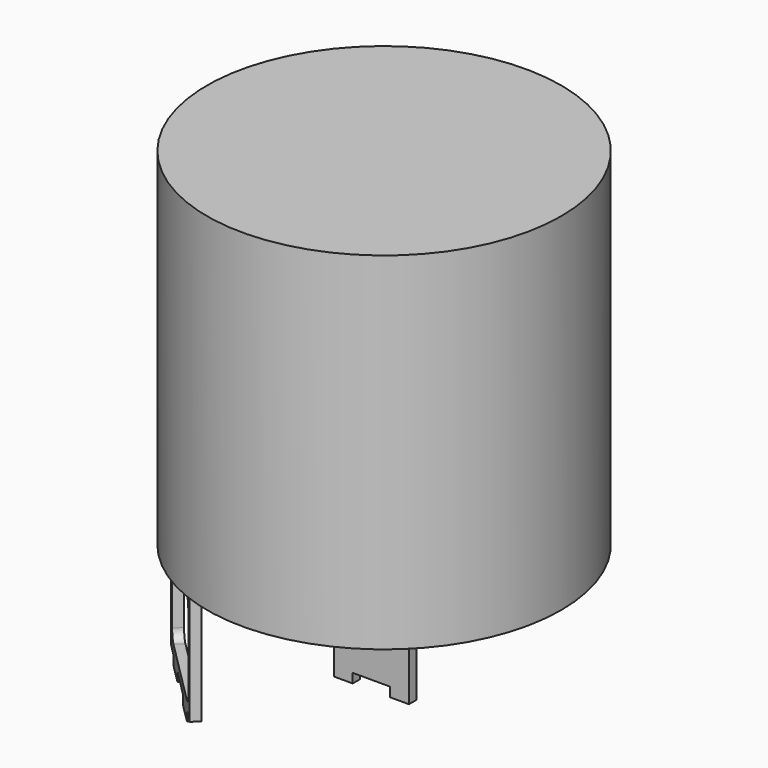
from build123d import *

# Parameters (mm, degrees)
F0_R     = 240
F1_DEPTH = 470
F2_R     = 3.175
F2_W     = 25.4
F2_H     = 12.7
F2_R_2   = 44.45
F3_DEPTH = 12.7
F4_W     = 38.1
F4_H     = 12.7
F5_DEPTH = 12.7
F6_R     = 3.175
F7_DEPTH = 12.7


# Not quite as in the source:
# - a feature names something its author has since deleted; it is built from what else it names


with BuildPart() as f1:
    # F0 (on Top) → F1 (new body)
    with BuildSketch(Plane.XY):
        Circle(F0_R)
    extrude(amount=F1_DEPTH)


with BuildPart() as f3:
    # F2 (on Top) → F3 (new body)
    with BuildSketch(Plane.XY):
        Polygon((107.8911188479, 199.151177898), (89.9306066058, 217.1116901402), (-89.9306066058, 217.1116901402), (-107.8911188479, 199.151177898), (-98.9108627269, 190.1709217769), (-125.8516310901, 163.2301534137), (-134.8318872111, 172.2104095348), (-172.2104095348, 134.8318872111), (-163.2301534137, 125.8516310901), (-190.1709217769, 98.9108627269), (-199.151177898, 107.8911188479), (-217.1116901402, 89.9306066058), (-217.1116901402, -89.9306066058), (-199.151177898, -107.8911188479), (-190.1709217769, -98.9108627269), (-163.2301534137, -125.8516310901), (-172.2104095348, -134.8318872111), (-134.8318872111, -172.2104095348), (-125.8516310901, -163.2301534137), (-98.9108627269, -190.1709217769), (-107.8911188479, -199.151177898), (-89.9306066058, -217.1116901402), (89.9306066058, -217.1116901402), (107.8911188479, -199.151177898), (98.9108627269, -190.1709217769), (125.8516310901, -163.2301534137), (134.8318872111, -172.2104095348), (172.2104095348, -134.8318872111), (163.2301534137, -125.8516310901), (190.1709217769, -98.9108627269), (199.151177898, -107.8911188479), (217.1116901402, -89.9306066058), (217.1116901402, 89.9306066058), (199.151177898, 107.8911188479), (190.1709217769, 98.9108627269), (163.2301534137, 125.8516310901), (172.2104095348, 134.8318872111), (134.8318872111, 172.2104095348), (125.8516310901, 163.2301534137), (98.9108627269, 190.1709217769), align=None)
        Polygon((-204.4116901402, -66.7095821215), (-204.4116901402, 66.7095821215), (-159.4195821215, 111.7016901402), (-60.6675371528, 111.7016901402), (-47.9675371528, 111.7016901402), (47.9675371528, 111.7016901402), (60.6675371528, 111.7016901402), (159.4195821215, 111.7016901402), (204.4116901402, 66.7095821215), (204.4116901402, -66.7095821215), (66.7095821215, -204.4116901402), (29.473233968, -204.4116901402), (-29.473233968, -204.4116901402), (-66.7095821215, -204.4116901402), align=None, mode=Mode.SUBTRACT)
        with Locations((-73.5717139989, 125.793881411)):
            Circle(F2_R, mode=Mode.SUBTRACT)
        with Locations((-66.1282860011, 143.3294988693)):
            Circle(F2_R, mode=Mode.SUBTRACT)
        with BuildLine():
            ThreePointArc((-30.343759404, 118.0516901402), (-46.853759404, 134.5616901402), (-30.343759404, 151.0716901402))
            Line((-30.343759404, 151.0716901402), (35.57801324, 151.0716901402))
            ThreePointArc((35.57801324, 151.0716901402), (52.08801324, 134.5616901402), (35.57801324, 118.0516901402))
            Line((35.57801324, 118.0516901402), (-30.343759404, 118.0516901402))
        make_face(mode=Mode.SUBTRACT)
        with Locations((73.5717139989, 125.793881411)):
            Circle(F2_R, mode=Mode.SUBTRACT)
        with Locations((66.1282860011, 143.3294988693)):
            Circle(F2_R, mode=Mode.SUBTRACT)
        with BuildLine():
            ThreePointArc((61.4490698794, 204.4116901402), (66.3091494704, 203.444960203), (70.4293260004, 200.6919462612))
            Line((70.4293260004, 200.6919462612), (113.6995821215, 157.4216901402))
            Line((113.6995821215, 157.4216901402), (-113.6995821215, 157.4216901402))
            Line((-113.6995821215, 157.4216901402), (-70.4293260004, 200.6919462612))
            ThreePointArc((-70.4293260004, 200.6919462612), (-66.3091494704, 203.444960203), (-61.4490698794, 204.4116901402))
            Line((-61.4490698794, 204.4116901402), (61.4490698794, 204.4116901402))
        make_face(mode=Mode.SUBTRACT)
        with BuildLine():
            Line((-47.9675371528, 111.7016901402), (-60.6675371528, 111.7016901402))
            Line((-60.6675371528, 111.7016901402), (-60.6675371528, -41.5995694615))
            ThreePointArc((-60.6675371528, -41.5995694615), (-52.9833960385, -90.0931268942), (-29.473233968, -133.1969946623))
            Line((-29.473233968, -133.1969946623), (-29.473233968, -204.4116901402))
            Line((-29.473233968, -204.4116901402), (29.473233968, -204.4116901402))
            Line((29.473233968, -204.4116901402), (29.473233968, -133.1969946623))
            ThreePointArc((29.473233968, -133.1969946623), (52.9833960385, -90.0931268942), (60.6675371528, -41.5995694615))
            Line((60.6675371528, -41.5995694615), (60.6675371528, 111.7016901402))
            Line((60.6675371528, 111.7016901402), (47.9675371528, 111.7016901402))
            Line((47.9675371528, 111.7016901402), (47.9675371528, 3.9363902736))
            Line((47.9675371528, 3.9363902736), (-47.9675371528, 3.9363902736))
            Line((-47.9675371528, 3.9363902736), (-47.9675371528, 111.7016901402))
        make_face()
        with Locations((-38.1, -15.1136097264)):
            Rectangle(F2_W, F2_H, mode=Mode.SUBTRACT)
        with Locations((0, -70.9936097264)):
            Circle(F2_R_2, mode=Mode.SUBTRACT)
        with Locations((38.1, -15.1136097264)):
            Rectangle(F2_W, F2_H, mode=Mode.SUBTRACT)
    extrude(amount=F3_DEPTH)


with BuildPart() as f5:
    # F4 (on face) → F5 (new body)
    with BuildSketch(Plane(origin=(-144.5408922519, -144.5408922519, 0), x_dir=(0.7071067812, -0.7071067812, 0), z_dir=(-0.7071067812, -0.7071067812, 0))):
        Polygon((-26.4306066058, 0), (-64.5306066058, 0), (-89.9306066058, 0), (-89.9306066058, -152.4), (-64.5306066058, -152.4), (-64.5306066058, -165.1), (-26.4306066058, -165.1), (-26.4306066058, -152.4), (26.4306066058, -152.4), (26.4306066058, -165.1), (64.5306066058, -165.1), (64.5306066058, -152.4), (89.9306066058, -152.4), (89.9306066058, 0), (64.5306066058, 0), (64.5306066058, 12.7), (26.4306066058, 12.7), (26.4306066058, 0), align=None)
        with BuildLine():
            Line((-64.5306066058, -12.7), (64.5306066058, -12.7))
            ThreePointArc((64.5306066058, -12.7), (73.5108627269, -16.4197438789), (77.2306066058, -25.4))
            Line((77.2306066058, -25.4), (77.2306066058, -127))
            ThreePointArc((77.2306066058, -127), (73.5108627269, -135.9802561211), (64.5306066058, -139.7))
            Line((64.5306066058, -139.7), (-64.5306066058, -139.7))
            ThreePointArc((-64.5306066058, -139.7), (-73.5108627269, -135.9802561211), (-77.2306066058, -127))
            Line((-77.2306066058, -127), (-77.2306066058, -25.4))
            ThreePointArc((-77.2306066058, -25.4), (-73.5108627269, -16.4197438789), (-64.5306066058, -12.7))
        make_face(mode=Mode.SUBTRACT)
        with Locations((-45.4806066058, 6.35)):
            Rectangle(F4_W, F4_H)
    extrude(amount=F5_DEPTH)


with BuildPart() as f7:
    # F6 (on face) → F7 (new body)
    with BuildSketch(Plane.XZ.offset(8.7636097264)):
        Polygon((25.4, 0), (-25.4, 0), (-25.4, 12.7), (-50.8, 12.7), (-50.8, 0), (-50.8, -152.4), (-50.8, -165.1), (-25.4, -165.1), (-25.4, -152.4), (25.4, -152.4), (25.4, -165.1), (50.8, -165.1), (50.8, -152.4), (50.8, 0), (50.8, 12.7), (25.4, 12.7), align=None)
        with Locations((-9.525, -101.6)):
            Circle(F6_R, mode=Mode.SUBTRACT)
        with Locations((9.525, -101.6)):
            Circle(F6_R, mode=Mode.SUBTRACT)
        with Locations((0, -47.625)):
            Circle(F6_R, mode=Mode.SUBTRACT)
        with Locations((-9.525, -38.1)):
            Circle(F6_R, mode=Mode.SUBTRACT)
        with Locations((0, -28.575)):
            Circle(F6_R, mode=Mode.SUBTRACT)
        with Locations((9.525, -38.1)):
            Circle(F6_R, mode=Mode.SUBTRACT)
    extrude(amount=F7_DEPTH)


solid = Compound([f1.part, f3.part, f5.part, f7.part])
